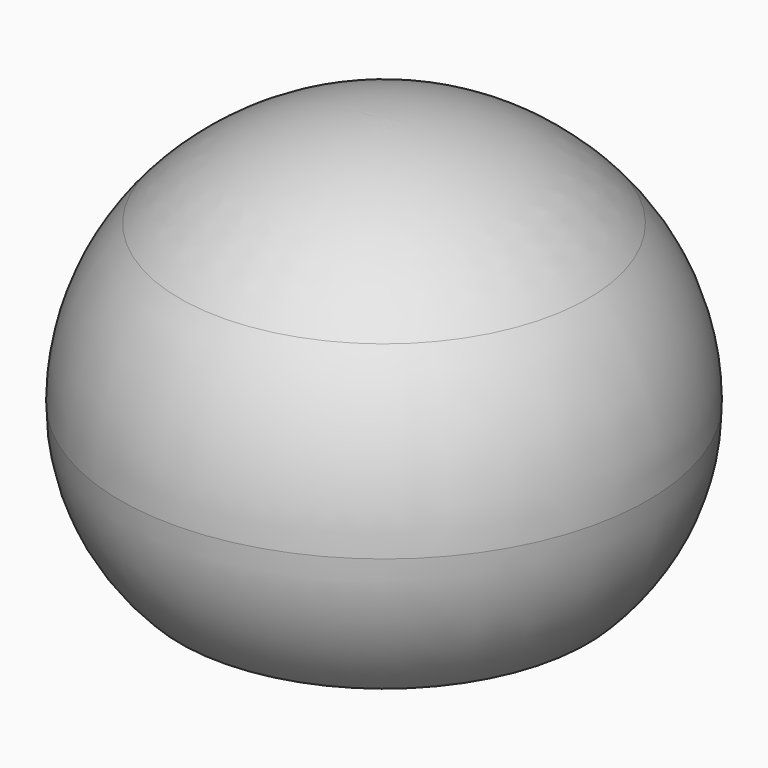
from build123d import *

# Parameters (mm, degrees)
F2_R = 1.2
F3_R = 1.5


# Not quite as in the source:
# - ends of sketch curves that miss each other by under 0.0002 mm in the source are joined


with BuildPart() as f1:
    # F0 (on Front) → F1 (revolve)
    with BuildSketch(Plane.XZ):
        with BuildLine():
            ThreePointArc((-3.15, 22.1655207886), (-3.905240004, 21.9827173041), (-4.65, 21.7610483486))
            Line((-4.65, 21.7610483486), (-4.65, 17.6655207886))
            Line((-4.65, 17.6655207886), (-3.15, 17.6655207886))
            Line((-3.15, 17.6655207886), (-3.15, 22.1655207886))
        make_face()
        with BuildLine():
            ThreePointArc((-11.2499970039, 17.4215708138), (-8.2407671062, 20.0335452886), (-4.65, 21.7610483486))
            ThreePointArc((-4.65, 21.7610483486), (-3.905240004, 21.9827173041), (-3.15, 22.1655207886))
            ThreePointArc((-3.15, 22.1655207886), (-1.583854187, 22.416145813), (0, 22.5))
            Line((0, 22.5), (0, 24))
            ThreePointArc((0, 24), (-6.7887220518, 22.5387255473), (-12.3749970039, 18.4137281594))
            ThreePointArc((-12.3749970039, 18.4137281594), (-15.0635072272, 13.9494024613), (-16, 8.8228761085))
            ThreePointArc((-16, 8.8228761085), (-15.0528039963, 4.0497512852), (-12.3547648239, 0))
            Line((-12.3547648239, 0), (-10.0693874848, 0))
            ThreePointArc((-10.0693874848, 0), (-13.3301386312, 3.8864435265), (-14.4999996005, 8.8228761085))
            ThreePointArc((-14.4999996005, 8.8228761085), (-13.6603854135, 13.4190720223), (-11.2499970039, 17.4215708138))
        make_face()
    revolve(axis=Axis((0, 0, 23.25), (0, 0, 1)))

    # F2
    f2_edges = [f1.edges().sort_by_distance(p)[0] for p in [
        (3.15, 0, 17.665521),
    ]]
    fillet(f2_edges, radius=F2_R)

    # F3
    f3_edges = [f1.edges().sort_by_distance(p)[0] for p in [
        (4.65, 0, 21.761048),
    ]]
    fillet(f3_edges, radius=F3_R)


solid = f1.part
